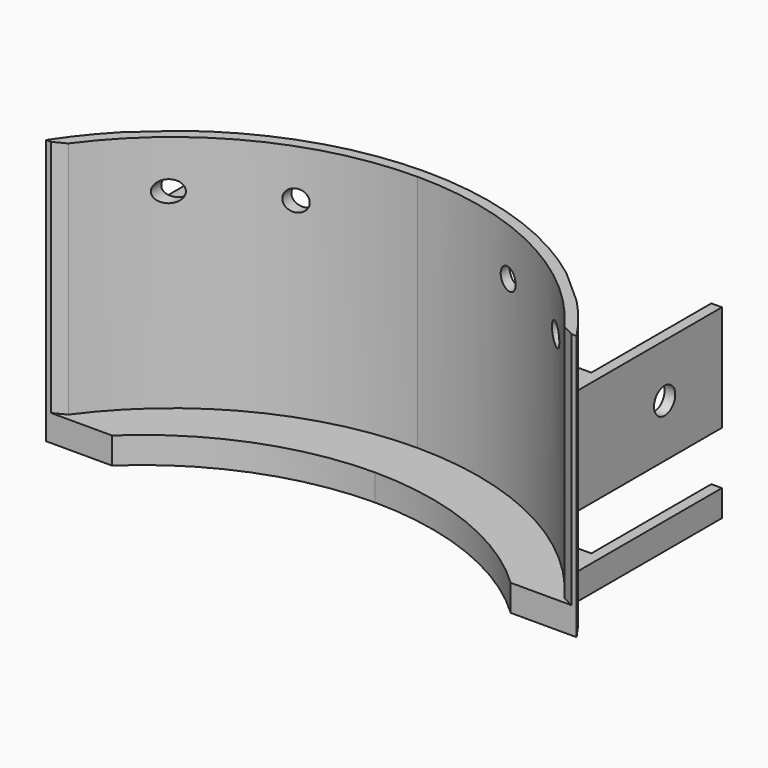
from build123d import *

# Parameters (mm, degrees)
F1_DEPTH    = 50
F3_DEPTH    = 15
F5_DEPTH    = 15
F6_R        = 2.5
F7_DEPTH    = 93.001
F8_T1_DEPTH = 57.6539038248
F9_DEPTH    = 5
F10_R       = 2
F11_DEPTH   = 33


# Not quite as in the source:
# - a fillet or chamfer that OpenCascade refuses, or shapes differently, is made with other operations: its cross-section is extruded or revolved along the edge and cut away or added


with BuildPart() as f1:
    # F0 (on Top) → F1 (new body)
    with BuildSketch(Plane.XY):
        with BuildLine():
            ThreePointArc((-43, 8.7560448021), (-46.7056429154, 4.5424231597), (-50, 0))
            Line((-50, 0), (-47.5900705485, 0))
            ThreePointArc((-47.5900705485, 0), (-26.8784989109, 18.3696900801), (0, 25))
            ThreePointArc((0, 25), (26.8784989109, 18.3696900801), (47.5900705485, 0))
            Line((47.5900705485, 0), (50, 0))
            ThreePointArc((50, 0), (46.7056429154, 4.5424231597), (43, 8.7560448021))
            Line((43, 8.7560448021), (43, 43))
            Line((43, 43), (41, 43))
            Line((41, 43), (41, 14.7306729384))
            Line((41, 14.7306729384), (36.2875219066, 14.7306729384))
            ThreePointArc((36.2875219066, 14.7306729384), (0, 27), (-36.2875219066, 14.7306729384))
            Line((-36.2875219066, 14.7306729384), (-41, 14.7306729384))
            Line((-41, 14.7306729384), (-41, 43))
            Line((-41, 43), (-43, 43))
            Line((-43, 43), (-43, 8.7560448021))
        make_face()
    extrude(amount=F1_DEPTH)

    # F2 (on face) → F3 (cut)
    with BuildSketch(Plane.XY.offset(50)):
        Polygon((-43, 8.7560448021), (-36.2875219066, 14.7306729384), (-41, 14.7306729384), (-41, 43), (-43, 43), align=None)
        Polygon((41, 43), (41, 14.7306729384), (36.2875219066, 14.7306729384), (43, 8.7560448021), (43, 43), align=None)
    extrude(amount=-F3_DEPTH, mode=Mode.SUBTRACT)

    # F4 (on face) → F5 (cut)
    with BuildSketch(Plane(origin=(0, 0, 0), x_dir=(1, 0, 0), z_dir=(0, 0, -1))):
        Polygon((-36.2875219066, -14.7306729384), (-43, -8.7560448021), (-43, -43), (-41, -43), (-41, -14.7306729384), align=None)
        Polygon((43, -8.7560448021), (36.2875219066, -14.7306729384), (41, -14.7306729384), (41, -43), (43, -43), align=None)
    extrude(amount=-F5_DEPTH, mode=Mode.SUBTRACT)

    # F6 (on face) → F7 (cut, through all)
    with BuildSketch(Plane(origin=(-43, 0, 0), x_dir=(0, -1, 0), z_dir=(-1, 0, 0))):
        with Locations((-29.5, 25)):
            Circle(F6_R)
    extrude(amount=-F7_DEPTH, mode=Mode.SUBTRACT)

    # F8: chamfer of 1.5 on 2 edges, made by hand

    # F8_s2 → F8_t1 (cut)
    with BuildSketch(Plane.XY.offset(-3.8269519124)):
        with BuildLine():
            Line((-49.1206089535, -0.027238599), (-46.7036689522, 1.2042065191))
            Line((-46.7036689522, 1.2042065191), (-46.6793989906, 1.186572207))
            ThreePointArc((-46.6793989906, 1.186572207), (-47.1374385844, 0.5954223102), (-47.565368237, -0.0170233899))
            Line((-47.565368237, -0.0170233899), (-47.5900705485, -0.03))
            ThreePointArc((-47.5900705485, -0.03), (-48.355339751, -0.03), (-49.1206089535, -0.057238599))
            Line((-49.1206089535, -0.057238599), (-49.1206089535, -0.027238599))
        make_face()
        with BuildLine():
            Line((46.7036689522, 1.2042065191), (49.1206089535, -0.027238599))
            Line((49.1206089535, -0.027238599), (49.1206089535, -0.057238599))
            ThreePointArc((49.1206089535, -0.057238599), (48.355339751, -0.03), (47.5900705485, -0.03))
            Line((47.5900705485, -0.03), (47.565368237, -0.0170233899))
            ThreePointArc((47.565368237, -0.0170233899), (47.1374385844, 0.5954223102), (46.6793989906, 1.186572207))
            Line((46.6793989906, 1.186572207), (46.7036689522, 1.2042065191))
        make_face()
    extrude(amount=F8_T1_DEPTH, mode=Mode.SUBTRACT)

    # F0 (on Top) → F9 (join)
    with BuildSketch(Plane.XY):
        with BuildLine():
            ThreePointArc((-43, 8.7560448021), (-46.7056429154, 4.5424231597), (-50, 0))
            Line((-50, 0), (-47.5900705485, 0))
            ThreePointArc((-47.5900705485, 0), (-26.8784989109, 18.3696900801), (0, 25))
            ThreePointArc((0, 25), (26.8784989109, 18.3696900801), (47.5900705485, 0))
            Line((47.5900705485, 0), (50, 0))
            ThreePointArc((50, 0), (46.7056429154, 4.5424231597), (43, 8.7560448021))
            Line((43, 8.7560448021), (43, 43))
            Line((43, 43), (41, 43))
            Line((41, 43), (41, 14.7306729384))
            Line((41, 14.7306729384), (36.2875219066, 14.7306729384))
            ThreePointArc((36.2875219066, 14.7306729384), (0, 27), (-36.2875219066, 14.7306729384))
            Line((-36.2875219066, 14.7306729384), (-41, 14.7306729384))
            Line((-41, 14.7306729384), (-41, 43))
            Line((-41, 43), (-43, 43))
            Line((-43, 43), (-43, 8.7560448021))
        make_face()
        with BuildLine():
            ThreePointArc((0, 25), (-26.8784989109, 18.3696900801), (-47.5900705485, 0))
            Line((-47.5900705485, 0), (-37.5900705485, 0))
            ThreePointArc((-37.5900705485, 0), (-20.2249265861, 11.0833143525), (0, 15))
            Line((0, 15), (0, 25))
        make_face()
        with BuildLine():
            ThreePointArc((47.5900705485, 0), (26.8784989109, 18.3696900801), (0, 25))
            Line((0, 25), (0, 15))
            ThreePointArc((0, 15), (20.2249265861, 11.0833143525), (37.5900705485, 0))
            Line((37.5900705485, 0), (47.5900705485, 0))
        make_face()
    extrude(amount=F9_DEPTH)

    # F10 (on Front) → F11 (cut)
    with BuildSketch(Plane.XZ):
        with Locations((-36.5, 41)):
            Circle(F10_R)
        with Locations((-20, 41)):
            Circle(F10_R)
        with Locations((20, 41)):
            Circle(F10_R)
        with Locations((36.5, 41)):
            Circle(F10_R)
    extrude(amount=-F11_DEPTH, mode=Mode.SUBTRACT)


solid = f1.part
